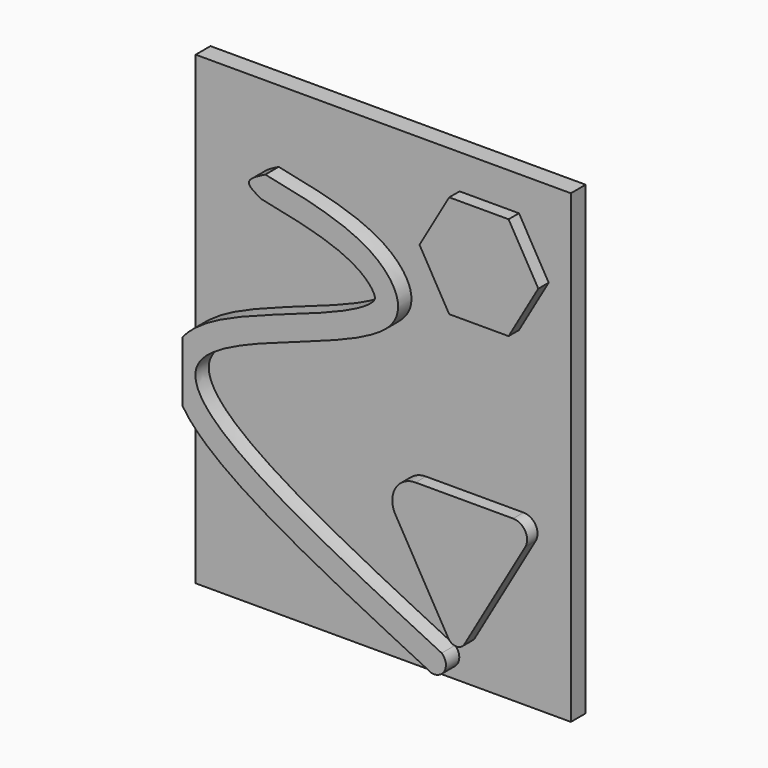
from build123d import *

# Parameters (mm, degrees)
F0_W     = 102.7496866882
F0_H     = 127.4545267224
F1_DEPTH = 5.08
F3_DEPTH = 4.572
F5_DEPTH = 3.556


# Not quite as in the source:
# - the dataset's text gives a spline's control points without its knots; the knots are read off the source's solid


with BuildPart() as f1:
    # F0 (on Front) → F1 (new body)
    with BuildSketch(Plane.XZ):
        with Locations((-12.3524237424, -0.9825788438)):
            Rectangle(F0_W, F0_H)
    extrude(amount=F1_DEPTH)

    # F2 (on face) → F3 (join)
    with BuildSketch(Plane.XZ.offset(5.08)):
        with BuildLine():
            add(Edge.make_bspline(
                [(-40.9875810146, 43.0931076407), (-28.9754866513, 40.6541317439), (-8.9047199794, 36.5788960137), (2.6934117166, 11.0659930573), (-97.3720869701, -5.2363998443), (-29.5336382259, -38.5052144585), (7.2991582565, -56.5684735775)],
                knots=[0, 0, 0, 0, 0.2185028084, 0.3650919442, 0.6552775065, 1, 1, 1, 1], degree=3))
            add(Edge.make_bspline(
                [(-42.2511235626, 36.8700890622), (-43.8847010474, 37.8139253556), (-47.3829993536, 39.8351462266), (-43.211266863, 41.9603150216), (-40.9875810146, 43.0931076407)],
                knots=[0, 0, 0, 0, 0.466963461, 1, 1, 1, 1], degree=3))
            add(Edge.make_bspline(
                [(-42.2511235626, 36.8700890622), (-40.5331687611, 36.5212697617), (-37.1284263592, 35.8298377024), (-32.2037648825, 34.7504733208), (-27.557338322, 33.5748117681), (-23.2917558848, 32.2586886151), (-19.5140115661, 30.7736402289), (-16.8597412875, 29.3923527839), (-15.0688958787, 28.2133967193), (-13.8956119979, 27.2981985917), (-12.8841109644, 26.3494674432), (-12.0705289044, 25.412010608), (-11.4857225122, 24.547708187), (-11.1367827325, 23.8262971232), (-10.9927915968, 23.3127055017), (-10.9753773189, 23.0245537892), (-10.9973004694, 22.8705191851), (-11.0567092302, 22.6874676103), (-11.2074929017, 22.4246551957), (-11.3671185487, 22.2063060575), (-11.5463278917, 21.9987612528), (-11.7628046407, 21.7708522191), (-12.1377373521, 21.4224331427), (-12.7473061949, 20.9360870019), (-13.7622136514, 20.2227466426), (-15.3804005447, 19.250355887), (-17.7862273921, 18.027148183), (-21.4973395358, 16.3638205241), (-26.8848647518, 14.2634749573), (-34.0118382966, 11.7253904926), (-40.1116945101, 9.5607985734), (-44.8763355502, 7.7634940467), (-48.3448392867, 6.3693900641), (-51.664785794, 4.9118983493), (-54.7992224423, 3.3656510124), (-57.7193061657, 1.6899577614), (-59.9581186489, 0.128235845), (-61.6203198311, -1.285228489), (-62.7435784588, -2.4016723909), (-63.4248349948, -3.2092037634), (-63.7272670865, -3.6053296012)],
                knots=[0, 0, 0, 0, 0.03125, 0.0625, 0.09375, 0.125, 0.15625, 0.1875, 0.203125, 0.21875, 0.234375, 0.25, 0.265625, 0.28125, 0.296875, 0.3125, 0.328125, 0.34375, 0.3515625, 0.359375, 0.36328125, 0.3671875, 0.375, 0.3828125, 0.390625, 0.40625, 0.421875, 0.4375, 0.46875, 0.5, 0.53125, 0.546875, 0.5625, 0.578125, 0.59375, 0.609375, 0.625, 0.6328125, 0.640625, 0.647416384, 0.647416384, 0.647416384, 0.647416384], degree=3))
            Line((-63.7272670865, -3.6053296012), (-63.7272670865, -19.9997841481))
            add(Edge.make_bspline(
                [(-63.7272670865, -19.9997841481), (-63.4472635638, -20.4353637772), (-62.5392656874, -21.7461458238), (-60.8020917377, -23.8282261522), (-58.3828342101, -26.2417888707), (-54.7531151656, -29.390420274), (-49.4898878144, -33.2771098209), (-42.1318250411, -37.9757896916), (-33.8817790935, -42.7375780579), (-24.9090488439, -47.563770943), (-15.3941700922, -52.4416603814), (-5.5244250361, -57.3521468944), (1.1641759191, -60.6323007913), (4.5031657206, -62.2697827025)],
                knots=[0.7268452432, 0.7268452432, 0.7268452432, 0.7268452432, 0.734375, 0.75, 0.765625, 0.78125, 0.8125, 0.84375, 0.875, 0.90625, 0.9375, 0.96875, 1, 1, 1, 1], degree=3))
            ThreePointArc((4.5031657206, -62.2697827025), (8.1339112347, -60.5140959957), (7.2991582565, -56.5684735775))
        make_face()
    extrude(amount=F3_DEPTH)

    # F4 (on face) → F5 (join)
    with BuildSketch(Plane.XZ.offset(5.08)):
        with BuildLine():
            Line((26.0450972097, -18.4491379124), (-0.6788218925, -18.4491379124))
            ThreePointArc((-0.6788218925, -18.4491379124), (-6.1780832066, -21.6241379124), (-6.1780832066, -27.9741379124))
            Line((-6.1780832066, -27.9741379124), (8.3186144479, -53.0831547919))
            ThreePointArc((8.3186144479, -53.0831547919), (10.5183189735, -54.3531547919), (12.7180234991, -53.0831547919))
            Line((12.7180234991, -53.0831547919), (29.3795398386, -24.2245619607))
            ThreePointArc((29.3795398386, -24.2245619607), (29.3795398386, -20.3742792618), (26.0450972097, -18.4491379124))
        make_face()
        Polygon((8.5503183743, 25.1236557961), (24.8167901793, 25.1236557961), (32.9500260818, 39.2108336091), (24.8167901793, 53.2980114222), (8.5503183743, 53.2980114222), (0.4170824718, 39.2108336091), align=None)
    extrude(amount=F5_DEPTH)


solid = f1.part
